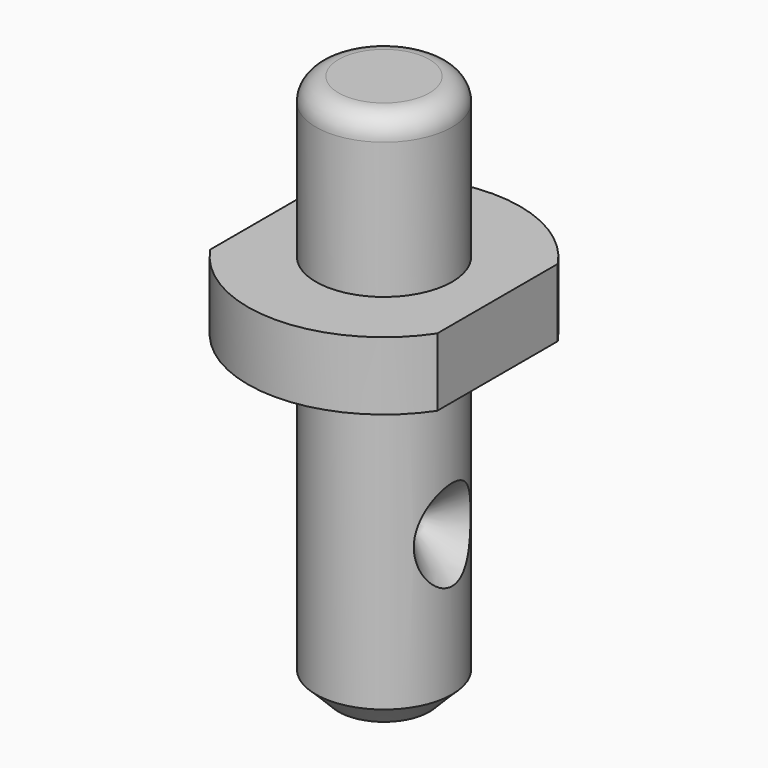
from build123d import *

# Parameters (mm, degrees)
F0_R     = 3
F1_DEPTH = 14
F3_DEPTH = 3
F4_R     = 3
F5_DEPTH = 7
F6_R     = 1
F8_R     = 2
F10_SIZE = 1


# Not quite as in the source:
# - an extrude whose draft closes it to a point is written as a loft to that point


with BuildPart() as f1:
    # F0 (on Top) → F1 (new body)
    with BuildSketch(Plane.XY):
        Circle(F0_R)
    extrude(amount=F1_DEPTH)

    # F2 (on face) → F3 (join)
    with BuildSketch(Plane.XY.offset(14)):
        with BuildLine():
            Line((-5, 3.3166247904), (-5, -3.3166247904))
            ThreePointArc((-5, -3.3166247904), (0, -6), (5, -3.3166247904))
            Line((5, -3.3166247904), (5, 3.3166247904))
            ThreePointArc((5, 3.3166247904), (0, 6), (-5, 3.3166247904))
        make_face()
    extrude(amount=F3_DEPTH)

    # F4 (on face) → F5 (join)
    with BuildSketch(Plane.XY.offset(17)):
        Circle(F4_R)
    extrude(amount=F5_DEPTH)

    # F6
    f6_edges = [f1.edges().sort_by_distance(p)[0] for p in [
        (-3, 0, 24),
    ]]
    fillet(f6_edges, radius=F6_R)

    # F8 (on offset) → F9 section 0
    with BuildSketch(Plane.YZ.offset(3), mode=Mode.PRIVATE) as f9_s0:
        with Locations((0, 7.2)):
            Circle(F8_R)
    loft([f9_s0.sketch, Vertex(1, 0, 7.2)], ruled=True, mode=Mode.SUBTRACT)

    # F10
    f10_edges = [f1.edges().sort_by_distance(p)[0] for p in [
        (-3, 0, 0),
    ]]
    chamfer(f10_edges, length=F10_SIZE)


solid = f1.part
